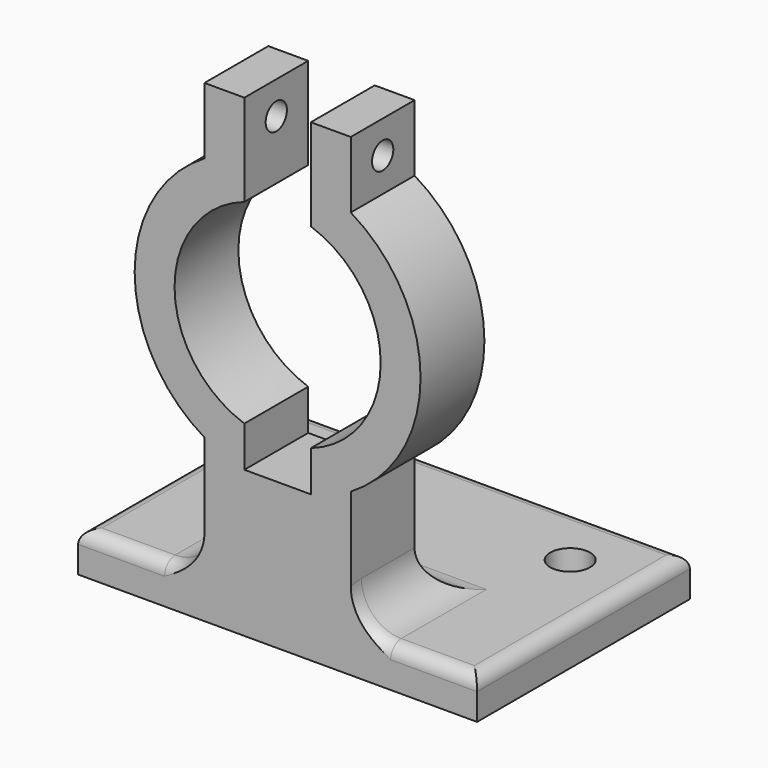
from build123d import *

# Parameters (mm, degrees)
F1_DEPTH      = 6
F2_R          = 1
F3_DEPTH      = 25
F5_DEPTH      = 6
F6_DEPTH      = 10
F11_R         = 1
F12_T1_DEPTH  = 5
F12_T3_DEPTH  = 11
F12_T8_ANGLE  = 359.64
F12_T14_ANGLE = 359.64
F12_T21_DEPTH = 12.5
F12_T25_DEPTH = 18.5
F12_T32_DEPTH = 18.5
F12_T36_DEPTH = 12.5
F13_R         = 1.5
F14_DEPTH     = 25


# Not quite as in the source:
# - a fillet or chamfer that OpenCascade refuses, or shapes differently, is made with other operations: its cross-section is extruded or revolved along the edge and cut away or added


with BuildPart() as f1:
    # F0 (on Front) → F1 (new body)
    with BuildSketch(Plane.XZ):
        with BuildLine():
            Line((2.5, -7.3357003756), (2.5, -18.4552618332))
            Line((2.5, -18.4552618332), (5.5, -18.4552618332))
            Line((5.5, -18.4552618332), (5.5, -9.236476601))
            ThreePointArc((5.5, -9.236476601), (10.75, 0), (5.5, 9.236476601))
            Line((5.5, 9.236476601), (5.5, 14.236476601))
            Line((5.5, 14.236476601), (2.5, 14.236476601))
            Line((2.5, 14.236476601), (2.5, 7.3357003756))
            ThreePointArc((2.5, 7.3357003756), (7.75, 0), (2.5, -7.3357003756))
        make_face()
    extrude(amount=F1_DEPTH)


with BuildPart() as f1b:
    # F0 (on Front) → F1, piece 2 (new body)
    with BuildSketch(Plane.XZ):
        with BuildLine():
            ThreePointArc((-2.5, -7.3357003756), (-7.75, 0), (-2.5, 7.3357003756))
            Line((-2.5, 7.3357003756), (-2.5, 14.236476601))
            Line((-2.5, 14.236476601), (-5.5, 14.236476601))
            Line((-5.5, 14.236476601), (-5.5, 9.236476601))
            ThreePointArc((-5.5, 9.236476601), (-10.75, 0), (-5.5, -9.236476601))
            Line((-5.5, -9.236476601), (-5.5, -18.4552618332))
            Line((-5.5, -18.4552618332), (-2.5, -18.4552618332))
            Line((-2.5, -18.4552618332), (-2.5, -7.3357003756))
        make_face()
    extrude(amount=F1_DEPTH)


with BuildPart() as f3_tool:
    # F2 (on face) → F3 (new body)
    with BuildSketch(Plane.YZ.offset(5.5)):
        with Locations((-3, 11.7896459997)):
            Circle(F2_R)
    extrude(amount=-F3_DEPTH)


with BuildPart() as f1_1:
    add(f1.part)

    # F3: cut by f3_tool
    add(f3_tool.part, mode=Mode.SUBTRACT)


with BuildPart() as f1b_1:
    add(f1b.part)

    # F3: cut by f3_tool
    add(f3_tool.part, mode=Mode.SUBTRACT)


with BuildPart() as f5:
    # F4 (on Front) → F5 (new body)
    with BuildSketch(Plane.XZ):
        Polygon((2.5, -12.8954811044), (-2.5, -12.8954811044), (-2.5, -18.4552618332), (-2.5, -20.8968445659), (2.5, -20.8968445659), (2.5, -18.4552618332), align=None)
    extrude(amount=F5_DEPTH)


with BuildPart() as f6:
    # F4 (on Front) → F6 (new body, symmetric)
    with BuildSketch(Plane.XZ):
        Polygon((2.5, -20.8968445659), (-2.5, -20.8968445659), (-15, -20.8968445659), (-15, -23.8968445659), (15, -23.8968445659), (15, -20.8968445659), align=None)
    extrude(amount=F6_DEPTH, both=True)


with BuildPart() as f6_1:
    # F7: moved
    add(f6.part.moved(Location((0, 0, 2.5))))


with BuildPart() as f5_1:
    # F7: moved
    add(f5.part.moved(Location((0, 0, 2.5))))


with BuildPart() as f6_2:
    # F8: moved
    add(f6_1.part.moved(Location((0, 4, 0))))


with BuildPart() as f5_2:
    add(f5_1.part)

    # F9: union F6
    add(f6_2.part)

    # F10: union F1, F1b
    add(f1_1.part)
    add(f1b_1.part)

    # F11
    f11_edges = [f5_2.edges().sort_by_distance(p)[0] for p in [
        (-10.25, -6, -18.396845),
        (10.25, -6, -18.396845),
        (15, 4, -18.396845),
        (0, 14, -18.396845),
        (-15, 4, -18.396845),
    ]]
    fillet(f11_edges, radius=F11_R)

    # F12: fillet of radius 3 on 7 edges, made by hand

    # F12_s2 → F12_t1 (join)
    with BuildSketch(Plane.XZ):
        with BuildLine():
            ThreePointArc((-8.5, -18.3968445659), (-6.3786796564, -17.5181649094), (-5.5, -15.3968445659))
            Line((-5.5, -15.3968445659), (-5.5, -18.3968445659))
            Line((-5.5, -18.3968445659), (-8.5, -18.3968445659))
        make_face()
        with BuildLine():
            ThreePointArc((8.5, -18.3968445659), (6.3786796564, -17.5181649094), (5.5, -15.3968445659))
            Line((5.5, -15.3968445659), (5.5, -18.3968445659))
            Line((5.5, -18.3968445659), (8.5, -18.3968445659))
        make_face()
    extrude(amount=F12_T1_DEPTH)

    # F12_s4 → F12_t3 (join)
    with BuildSketch(Plane.YZ.offset(-5.5)):
        with BuildLine():
            ThreePointArc((3, -18.3968445659), (0.8786796564, -17.5181649094), (0, -15.3968445659))
            Line((0, -15.3968445659), (0, -18.3968445659))
            Line((0, -18.3968445659), (3, -18.3968445659))
        make_face()
    extrude(amount=F12_T3_DEPTH)


with BuildPart() as f12_tool6:
    # F12_s7 → F12_t8 (revolve)
    with BuildSketch(Plane.XZ.offset(5)):
        with BuildLine():
            ThreePointArc((-8.5, -18.3968445659), (-6.3786796564, -17.5181649094), (-5.5, -15.3968445659))
            Line((-5.5, -15.3968445659), (-5.5, -18.3968445659))
            Line((-5.5, -18.3968445659), (-8.5, -18.3968445659))
        make_face()
    revolve(axis=Axis((-5.5, -5, -19.3968445659), (1, 0, 0)), revolution_arc=F12_T8_ANGLE)

    split(bisect_by=Plane.XZ.offset(6), keep=Keep.BOTTOM)

    split(bisect_by=Plane.XY.offset(-21.3968445659), keep=Keep.TOP)


with BuildPart() as f5_3:
    add(f5_2.part)

    # F12_t5: union F12_tool6
    add(f12_tool6.part)


with BuildPart() as f12_tool12:
    # F12_s13 → F12_t14 (revolve)
    with BuildSketch(Plane.XZ.offset(5)):
        with BuildLine():
            ThreePointArc((8.5, -18.3968445659), (6.3786796564, -17.5181649094), (5.5, -15.3968445659))
            Line((5.5, -15.3968445659), (5.5, -18.3968445659))
            Line((5.5, -18.3968445659), (8.5, -18.3968445659))
        make_face()
    revolve(axis=Axis((5.5, -5, -19.3968445659), (1, 0, 0)), revolution_arc=F12_T14_ANGLE)

    split(bisect_by=Plane.XZ.offset(6), keep=Keep.BOTTOM)

    split(bisect_by=Plane.XY.offset(-21.3968445659), keep=Keep.TOP)


with BuildPart() as f5_4:
    add(f5_3.part)

    # F12_t11: union F12_tool12
    add(f12_tool12.part)


with BuildPart() as f12_tool19:
    # F12_s20 → F12_t21 (new body)
    with BuildSketch(Plane.XZ.offset(5)):
        with BuildLine():
            ThreePointArc((-8.5, -18.3968445659), (-6.3786796564, -17.5181649094), (-5.5, -15.3968445659))
            Line((-5.5, -15.3968445659), (-5.5, -18.3968445659))
            Line((-5.5, -18.3968445659), (-8.5, -18.3968445659))
        make_face()
    extrude(amount=-F12_T21_DEPTH)

    split(bisect_by=Plane.XZ, keep=Keep.BOTTOM)


with BuildPart() as f12_tool23:
    # F12_s24 → F12_t25 (new body)
    with BuildSketch(Plane.YZ.offset(-13)):
        with BuildLine():
            ThreePointArc((3, -18.3968445659), (0.8786796564, -17.5181649094), (0, -15.3968445659))
            Line((0, -15.3968445659), (0, -18.3968445659))
            Line((0, -18.3968445659), (3, -18.3968445659))
        make_face()
    extrude(amount=F12_T25_DEPTH)

    split(bisect_by=Plane.YZ.offset(-5.5), keep=Keep.BOTTOM)


with BuildPart() as f12_tool19_1:
    add(f12_tool19.part)

    # F12_t27: intersect F12_tool23
    add(f12_tool23.part, mode=Mode.INTERSECT)


with BuildPart() as f5_5:
    add(f5_4.part)

    # F12_t17: union F12_tool19
    add(f12_tool19_1.part)


with BuildPart() as f12_tool30:
    # F12_s31 → F12_t32 (new body)
    with BuildSketch(Plane.YZ.offset(-5.5)):
        with BuildLine():
            ThreePointArc((3, -18.3968445659), (0.8786796564, -17.5181649094), (0, -15.3968445659))
            Line((0, -15.3968445659), (0, -18.3968445659))
            Line((0, -18.3968445659), (3, -18.3968445659))
        make_face()
    extrude(amount=F12_T32_DEPTH)

    split(bisect_by=Plane.YZ.offset(5.5), keep=Keep.TOP)


with BuildPart() as f12_tool34:
    # F12_s35 → F12_t36 (new body)
    with BuildSketch(Plane.XZ.offset(-7.5)):
        with BuildLine():
            ThreePointArc((8.5, -18.3968445659), (6.3786796564, -17.5181649094), (5.5, -15.3968445659))
            Line((5.5, -15.3968445659), (5.5, -18.3968445659))
            Line((5.5, -18.3968445659), (8.5, -18.3968445659))
        make_face()
    extrude(amount=F12_T36_DEPTH)

    split(bisect_by=Plane.XZ, keep=Keep.BOTTOM)


with BuildPart() as f12_tool30_1:
    add(f12_tool30.part)

    # F12_t38: intersect F12_tool34
    add(f12_tool34.part, mode=Mode.INTERSECT)


with BuildPart() as f5_6:
    add(f5_5.part)

    # F12_t28: union F12_tool30
    add(f12_tool30_1.part)

    # F13 (on face) → F14 (cut)
    with BuildSketch(Plane.XY.offset(-18.3968445659)):
        with Locations((-10, 9)):
            Circle(F13_R)
        with Locations((10, 9)):
            Circle(F13_R)
    extrude(amount=-F14_DEPTH, mode=Mode.SUBTRACT)


solid = f5_6.part
